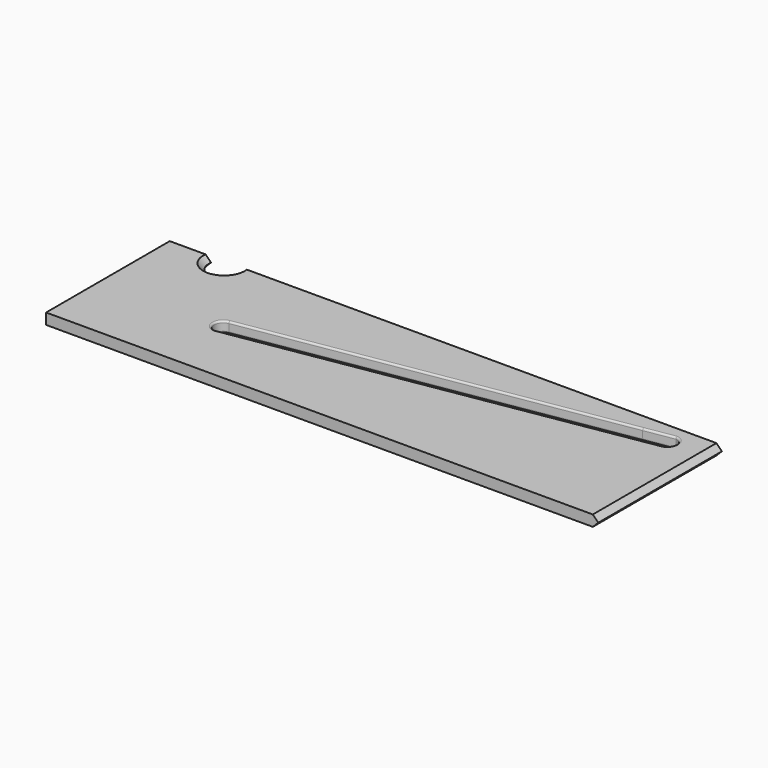
from build123d import *

# Parameters (mm, degrees)
F1_DEPTH    = 3
F2_T1_DEPTH = 52.6928029293
F2_T4_ANGLE = 359.64
F2_T6_ANGLE = 359.64
F3_R        = 0.5


# Not quite as in the source:
# - a fillet or chamfer that OpenCascade refuses, or shapes differently, is made with other operations: its cross-section is extruded or revolved along the edge and cut away or added


with BuildPart() as f1:
    # F0 (on Top) → F1 (new body)
    with BuildSketch(Plane.XY):
        with BuildLine():
            Line((0, -21.2030354887), (0, 0))
            Line((0, 0), (-18.5486488044, 0))
            Line((-18.5486488044, 0), (-18.5486488044, -4.6107494656))
            Line((-18.5486488044, -4.6107494656), (-10.5158546939, -3.2809847035))
            ThreePointArc((-10.5158546939, -3.2809847035), (-8.3883004552, -5.7297930738), (-10.4765901342, -8.212170098))
            Line((-10.4765901342, -8.212170098), (-18.5486488044, -9.5484347937))
            Line((-18.5486488044, -9.5484347937), (-18.5486488044, -21.2030354887))
            Line((-18.5486488044, -21.2030354887), (0, -21.2030354887))
        make_face()
        with BuildLine():
            Line((-18.5486488044, -4.6107494656), (-18.5486488044, 0))
            Line((-18.5486488044, 0), (-132.8552216291, 0))
            ThreePointArc((-132.8552216291, 0), (-136.5013867617, -4.4477159734), (-140.1475518942, 0))
            Line((-140.1475518942, 0), (-152.0042717457, 0))
            Line((-152.0042717457, 0), (-152.0042717457, -42.4060709774))
            Line((-152.0042717457, -42.4060709774), (0, -42.4060709774))
            Line((0, -42.4060709774), (0, -21.2030354887))
            Line((0, -21.2030354887), (-18.5486488044, -21.2030354887))
            Line((-18.5486488044, -21.2030354887), (-18.5486488044, -9.5484347937))
            Line((-18.5486488044, -9.5484347937), (-118.7394559383, -26.1342208833))
            ThreePointArc((-118.7394559383, -26.1342208833), (-120.8670101771, -23.6854125129), (-118.7787204981, -21.2030354887))
            Line((-118.7787204981, -21.2030354887), (-18.5486488044, -4.6107494656))
        make_face()
    extrude(amount=F1_DEPTH)

    # F2: chamfer of 2 on 4 edges, made by hand

    # F2_s2 → F2_t1 (cut)
    with BuildSketch(Plane.XZ.offset(-5.1433659759)):
        Polygon((0, 1), (-2, 3), (0, 3), align=None)
        Polygon((0, 2), (-2, 0), (0, 0), align=None)
    extrude(amount=F2_T1_DEPTH, mode=Mode.SUBTRACT)

    # F2_s3 → F2_t4 (revolve, cut)
    with BuildSketch(Plane(origin=(-136.4977483257, 0.4288217341, 0), x_dir=(0, 0, 1), z_dir=(-0.9999950652, 0.0031415875, 0))):
        Polygon((1, 2.5602393555), (3, 4.5602393555), (3, 2.5602393555), align=None)
    revolve(axis=Axis((-136.5013867617, -0.7293245843, 3), (0, 0, -1)), revolution_arc=F2_T4_ANGLE, mode=Mode.SUBTRACT)

    # F2_s5 → F2_t6 (revolve, cut)
    with BuildSketch(Plane(origin=(-136.4977483257, 0.4288217341, 0), x_dir=(0, 0, 1), z_dir=(-0.9999950652, 0.0031415875, 0))):
        Polygon((2, 2.5602393555), (0, 4.5602393555), (0, 2.5602393555), align=None)
    revolve(axis=Axis((-136.5013867617, -0.7293245843, 0), (0, 0, -1)), revolution_arc=F2_T6_ANGLE, mode=Mode.SUBTRACT)

    # F3
    f3_edges = [f1.edges().sort_by_distance(p)[0] for p in [
        (-64.647288, -12.24201, 3),
        (-64.608023, -17.173195, 3),
        (-120.86701, -23.685413, 3),
        (-8.3883, -5.729793, 3),
        (-64.647288, -12.24201, 0),
        (-8.3883, -5.729793, 0),
        (-120.86701, -23.685413, 0),
    ]]
    fillet(f3_edges, radius=F3_R)


solid = f1.part
